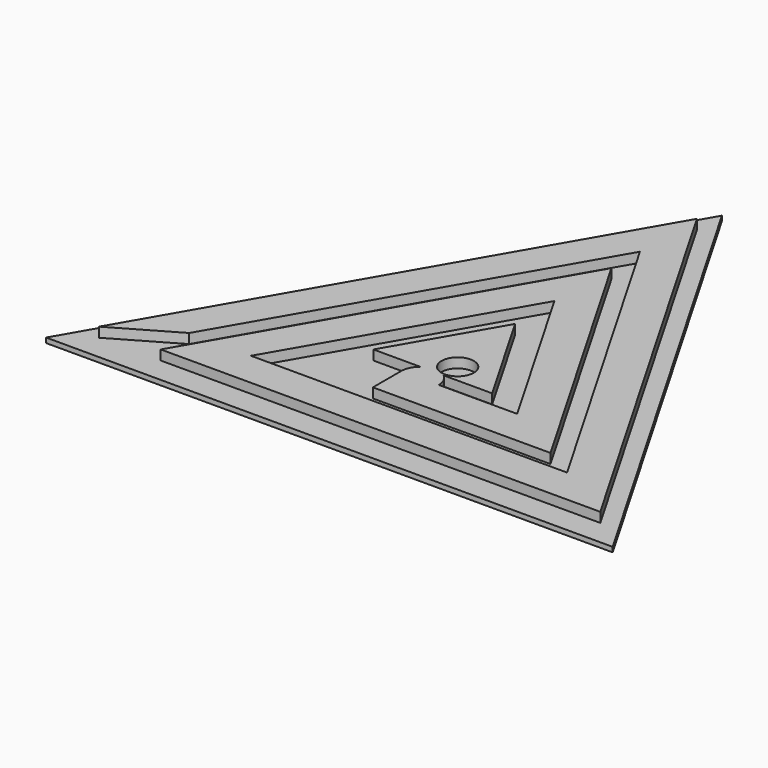
from build123d import *

# Parameters (mm, degrees)
F1_DEPTH = 5
F3_DEPTH = 10
F4_DEPTH = 10


# Not quite as in the source:
# - a feature names something its author has since deleted; it is built from what else it names


with BuildPart() as f1:
    # F0 (on Top) → F1 (new body)
    with BuildSketch(Plane.XY):
        Polygon((290, -167.431578065), (0, 334.86315613), (-290, -167.431578065), align=None)
    extrude(amount=F1_DEPTH)

    # F2 (on face) → F3 (join)
    with BuildSketch(Plane.XY.offset(5)):
        with BuildLine():
            Line((256.3882985588, -141.2744761391), (-0.1700333609, 303.0975898508))
            Line((-0.1700333609, 303.0975898508), (-256.7283652805, -141.2744761391))
            Line((-256.7283652805, -141.2744761391), (-193.5489429105, -104.7978196266))
            Line((-193.5489429105, -104.7978196266), (-0.1700333609, 230.1442768257))
            Line((-0.1700333609, 230.1442768257), (193.2088761888, -104.7978196266))
            Line((193.2088761888, -104.7978196266), (-130.3695205406, -104.7978196266))
            Line((-130.3695205406, -104.7978196266), (-0.1700333609, 120.7143072881))
            Line((-0.1700333609, 120.7143072881), (98.6142485835, -50.3850880286))
            Line((98.6142485835, -50.3850880286), (18.3761417155, -50.3850880286))
            ThreePointArc((18.3761417155, -50.3850880286), (16.3865094235, -41.8600549069), (10.8287170908, -35.0964929185))
            Line((10.8287170908, -35.0964929185), (-12.5935137719, -35.0964929185))
            ThreePointArc((-12.5935137719, -35.0964929185), (-18.1513061046, -41.8600549069), (-20.1409383966, -50.3850880286))
            Line((-20.1409383966, -50.3850880286), (-20.1409383966, -86.5594913703))
            Line((-20.1409383966, -86.5594913703), (161.6191650039, -86.5594913703))
            Line((161.6191650039, -86.5594913703), (-0.1700333609, 193.6676203132))
            Line((-0.1700333609, 193.6676203132), (-193.5489429105, -141.2744761391))
            Line((-193.5489429105, -141.2744761391), (256.3882985588, -141.2744761391))
        make_face()
    extrude(amount=F3_DEPTH)

    # F2 (on face) → F4 (join)
    with BuildSketch(Plane.XY.offset(5)):
        with BuildLine():
            Line((-60.7889089023, -35.0964929185), (-12.5935137719, -35.0964929185))
            ThreePointArc((-12.5935137719, -35.0964929185), (-7.065251394, -32.1460175148), (-0.8823983405, -31.1265479726))
            ThreePointArc((-0.8823983405, -31.1265479726), (1.9162643927, -31.3309847436), (4.6555093745, -31.9399547076))
            ThreePointArc((4.6555093745, -31.9399547076), (1.2463845952, -2.8955610808), (27.1223774556, -16.5202418624))
            ThreePointArc((27.1223774556, -16.5202418624), (20.4987699273, -29.7504111213), (5.9377581342, -32.3746235496))
            ThreePointArc((5.9377581342, -32.3746235496), (8.4826511964, -33.5569208004), (10.8287170908, -35.0964929185))
            Line((10.8287170908, -35.0964929185), (60.7889089023, -35.0964929185))
            Line((60.7889089023, -35.0964929185), (0, 70.1929858369))
            Line((0, 70.1929858369), (-60.7889089023, -35.0964929185))
        make_face()
        with BuildLine():
            ThreePointArc((-0.8823983405, -31.1265479726), (-7.065251394, -32.1460175148), (-12.5935137719, -35.0964929185))
            Line((-12.5935137719, -35.0964929185), (10.8287170908, -35.0964929185))
            ThreePointArc((10.8287170908, -35.0964929185), (8.4826511964, -33.5569208004), (5.9377581342, -32.3746235496))
            ThreePointArc((5.9377581342, -32.3746235496), (5.2921802317, -32.1704267711), (4.6555093745, -31.9399547076))
            ThreePointArc((4.6555093745, -31.9399547076), (1.9162643927, -31.3309847436), (-0.8823983405, -31.1265479726))
        make_face()
    extrude(amount=F4_DEPTH)


solid = f1.part
